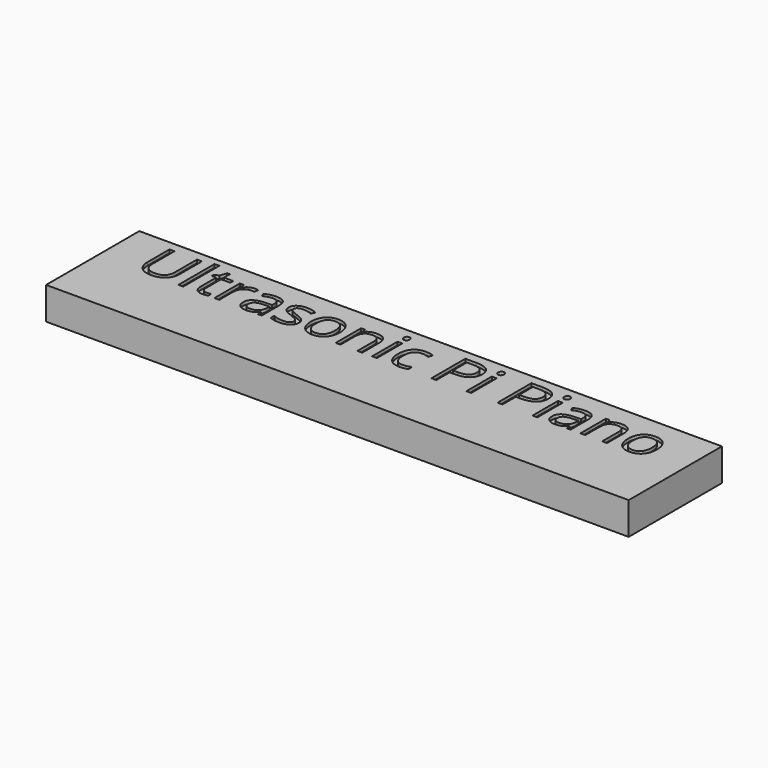
from build123d import *

# Parameters (mm, degrees)
F0_W         = 457.2
F0_H         = 91.44
F1_DEPTH     = 25.4
F2_TEXT_SIZE = 46.5288014311
F3_DEPTH     = 2.54


# Not quite as in the source:
# - Text() gives the source's letters only with a copy of the font that has no kerning and outlines rounded to 1/6400 em; it was checked with that copy


with BuildPart() as f1:
    # F0 (on Top) → F1 (new body)
    with BuildSketch(Plane.XY):
        with Locations((-228.6, -172.72)):
            Rectangle(F0_W, F0_H)
    extrude(amount=F1_DEPTH)

    # F2 (on face) → F3 (cut)
    with BuildSketch(Plane.XY.offset(25.4)):
        with Locations((-431.8, -167.64)):
            Text('Ultrasonic Pi Piano', F2_TEXT_SIZE, font='Open Sans', text_align=(TextAlign.LEFT, TextAlign.BOTTOM))
    extrude(amount=-F3_DEPTH, mode=Mode.SUBTRACT)


solid = f1.part
